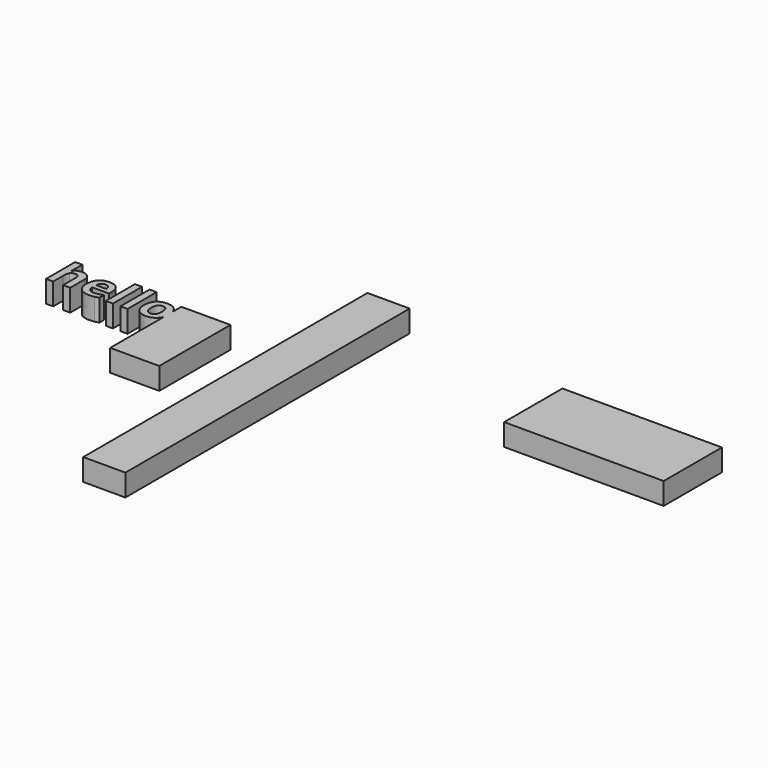
from build123d import *

# Parameters (mm, degrees)
F0_W     = 184.6868768334
F0_H     = 84.2627063394
F0_W_2   = 48.8200113177
F0_H_2   = 411.3924652338
F0_W_3   = 8.2527426776
F0_H_3   = 42.1123689836
F1_DEPTH = 25.4


with BuildPart() as f1:
    # F0 (on Top) → F1 (new body)
    with BuildSketch(Plane.XY):
        with Locations((184.7166828811, 123.0147741735)):
            Rectangle(F0_W, F0_H)
        with Locations((-137.6638747752, -4.5765265822)):
            Rectangle(F0_W_2, F0_H_2)
        with BuildLine():
            Line((-386.5573875373, 41.1865082052), (-378.3046448597, 41.1865082052))
            Line((-378.3046448597, 41.1865082052), (-378.3046448597, 60.9134209226))
            add(Edge.make_bspline(
                [(-381.0627755447, 69.1401843473), (-378.3046448597, 66.2738067751), (-378.3046448597, 60.9134209226)],
                knots=[0, 0, 0, 1, 1, 1], degree=2))
            add(Edge.make_bspline(
                [(-389.1553128293, 72.0065619195), (-383.8209062297, 72.0065619195), (-381.0627755447, 69.1401843473)],
                knots=[0, 0, 0, 1, 1, 1], degree=2))
            add(Edge.make_bspline(
                [(-397.9276405654, 67.5727694211), (-395.1651800049, 72.0065619195), (-389.1553128293, 72.0065619195)],
                knots=[0, 0, 0, 1, 1, 1], degree=2))
            Line((-397.9276405654, 67.5727694211), (-398.3606281141, 67.5727694211))
            Line((-398.3606281141, 67.5727694211), (-398.1701135926, 70.0061594447))
            add(Edge.make_bspline(
                [(-397.9795990712, 74.7170639742), (-397.9795990712, 73.7125328613), (-398.1701135926, 70.0061594447)],
                knots=[0, 0, 0, 1, 1, 1], degree=2))
            Line((-397.9795990712, 74.7170639742), (-397.9795990712, 83.2988771888))
            Line((-397.9795990712, 83.2988771888), (-406.2323417489, 83.2988771888))
            Line((-406.2323417489, 83.2988771888), (-406.2323417489, 41.1865082052))
            Line((-406.2323417489, 41.1865082052), (-397.9795990712, 41.1865082052))
            Line((-397.9795990712, 41.1865082052), (-397.9795990712, 55.4231388055))
            add(Edge.make_bspline(
                [(-396.438163398, 63.052379413), (-397.9795990712, 60.6969271483), (-397.9795990712, 55.4231388055)],
                knots=[0, 0, 0, 1, 1, 1], degree=2))
            add(Edge.make_bspline(
                [(-391.4328273353, 65.4078316778), (-394.8967277247, 65.4078316778), (-396.438163398, 63.052379413)],
                knots=[0, 0, 0, 1, 1, 1], degree=2))
            add(Edge.make_bspline(
                [(-386.5573875373, 58.8610599419), (-386.5573875373, 65.4078316778), (-391.4328273353, 65.4078316778)],
                knots=[0, 0, 0, 1, 1, 1], degree=2))
            Line((-386.5573875373, 58.8610599419), (-386.5573875373, 41.1865082052))
        make_face()
        Polygon((-336.9529306078, 41.1865082052), (-328.8141680467, 41.1865082052), (-328.8141680467, 83.2988771888), (-337.0669107244, 83.2988771888), (-337.0669107244, 41.1865082052), align=None)
        with Locations((-316.0280457345, 62.242692697)):
            Rectangle(F0_W_3, F0_H_3)
        with BuildLine():
            Line((-276.5679955482, 50.2645032945), (-276.5679955482, -28.1147938222))
            Line((-276.5679955482, -28.1147938222), (-219.7534025482, -28.1147938222))
            Line((-219.7534025482, -28.1147938222), (-219.7534025482, 74.9002173543))
            Line((-219.7534025482, 74.9002173543), (-276.5679955482, 74.9002173543))
            Line((-276.5679955482, 74.9002173543), (-276.5679955482, 62.2686307575))
            add(Edge.make_bspline(
                [(-276.5679955482, 62.2686307575), (-275.7472140818, 59.5977436271), (-275.7472140818, 56.3670516616)],
                knots=[0.3216911884, 0.3216911884, 0.3216911884, 1, 1, 1], degree=2))
            add(Edge.make_bspline(
                [(-275.7472140818, 56.3670516616), (-275.7472140818, 52.9769771283), (-276.5679955482, 50.2645032945)],
                knots=[0, 0, 0, 0.4589388385, 0.4589388385, 0.4589388385], degree=2))
        make_face()
        with BuildLine():
            add(Edge.make_bspline(
                [(-356.1183628659, 40.6409438939), (-363.4185329364, 40.6409438939), (-367.5319146488, 44.6763878475)],
                knots=[0, 0, 0, 1, 1, 1], degree=2))
            add(Edge.make_bspline(
                [(-350.1084956903, 41.1691887033), (-352.5678649668, 40.6409438939), (-356.1183628659, 40.6409438939)],
                knots=[0, 0, 0, 1, 1, 1], degree=2))
            add(Edge.make_bspline(
                [(-345.4841886705, 42.7799023843), (-347.6491264139, 41.6974335126), (-350.1084956903, 41.1691887033)],
                knots=[0, 0, 0, 1, 1, 1], degree=2))
            Line((-345.4841886705, 42.7799023843), (-345.4841886705, 49.1707986027))
            add(Edge.make_bspline(
                [(-350.5674624919, 47.3565807737), (-348.1340724684, 47.9237944625), (-345.4841886705, 49.1707986027)],
                knots=[0, 0, 0, 1, 1, 1], degree=2))
            add(Edge.make_bspline(
                [(-355.737333823, 46.789367085), (-353.0008525154, 46.789367085), (-350.5674624919, 47.3565807737)],
                knots=[0, 0, 0, 1, 1, 1], degree=2))
            add(Edge.make_bspline(
                [(-361.2016366872, 48.7637903069), (-359.2531927182, 46.789367085), (-355.737333823, 46.789367085)],
                knots=[0, 0, 0, 1, 1, 1], degree=2))
            add(Edge.make_bspline(
                [(-363.2886366718, 54.2540724241), (-363.1500806562, 50.7382135289), (-361.2016366872, 48.7637903069)],
                knots=[0, 0, 0, 1, 1, 1], degree=2))
            Line((-363.2886366718, 54.2540724241), (-343.7782177288, 54.2540724241))
            Line((-343.7782177288, 54.2540724241), (-343.7782177288, 58.2635371247))
            add(Edge.make_bspline(
                [(-347.3503650053, 68.3564768842), (-343.7782177288, 64.7063918489), (-343.7782177288, 58.2635371247)],
                knots=[0, 0, 0, 1, 1, 1], degree=2))
            add(Edge.make_bspline(
                [(-357.3307280021, 72.0065619195), (-350.9225122818, 72.0065619195), (-347.3503650053, 68.3564768842)],
                knots=[0, 0, 0, 1, 1, 1], degree=2))
            add(Edge.make_bspline(
                [(-367.8436656838, 67.8542113278), (-364.0420350065, 72.0065619195), (-357.3307280021, 72.0065619195)],
                knots=[0, 0, 0, 1, 1, 1], degree=2))
            add(Edge.make_bspline(
                [(-371.6452963611, 56.0985993814), (-371.6452963611, 63.701860736), (-367.8436656838, 67.8542113278)],
                knots=[0, 0, 0, 1, 1, 1], degree=2))
            add(Edge.make_bspline(
                [(-367.5319146488, 44.6763878475), (-371.6452963611, 48.7118318011), (-371.6452963611, 56.0985993814)],
                knots=[0, 0, 0, 1, 1, 1], degree=2))
        make_face()
        with BuildLine():
            add(Edge.make_bspline(
                [(-357.2787694963, 66.1352507595), (-359.9026740412, 66.1352507595), (-361.3921512086, 64.4725785727)],
                knots=[0, 0, 0, 1, 1, 1], degree=2))
            add(Edge.make_bspline(
                [(-353.1134292781, 64.4725785727), (-354.6548649513, 66.1352507595), (-357.2787694963, 66.1352507595)],
                knots=[0, 0, 0, 1, 1, 1], degree=2))
            add(Edge.make_bspline(
                [(-351.511375348, 59.7530142922), (-351.5719936048, 62.8099063858), (-353.1134292781, 64.4725785727)],
                knots=[0, 0, 0, 1, 1, 1], degree=2))
            Line((-351.511375348, 59.7530142922), (-363.0981221504, 59.7530142922))
            add(Edge.make_bspline(
                [(-361.3921512086, 64.4725785727), (-362.8816283761, 62.8099063858), (-363.0981221504, 59.7530142922)],
                knots=[0, 0, 0, 1, 1, 1], degree=2))
        make_face(mode=Mode.SUBTRACT)
        with BuildLine():
            add(Edge.make_bspline(
                [(-276.5679955482, 50.2645032945), (-277.5356473057, 47.0666605317), (-279.6441020198, 44.8106139876)],
                knots=[0.4589388385, 0.4589388385, 0.4589388385, 1, 1, 1], degree=2))
            Line((-276.5679955482, 50.2645032945), (-276.5679955482, 62.2686307575))
            add(Edge.make_bspline(
                [(-277.5311227823, 64.6760827205), (-276.9572550725, 63.5353117149), (-276.5679955482, 62.2686307575)],
                knots=[0, 0, 0, 0.3216911884, 0.3216911884, 0.3216911884], degree=2))
            add(Edge.make_bspline(
                [(-282.6447057321, 70.1144063318), (-279.3150314828, 68.2222507441), (-277.5311227823, 64.6760827205)],
                knots=[0, 0, 0, 1, 1, 1], degree=2))
            add(Edge.make_bspline(
                [(-290.330234721, 72.0065619195), (-285.9743799814, 72.0065619195), (-282.6447057321, 70.1144063318)],
                knots=[0, 0, 0, 1, 1, 1], degree=2))
            add(Edge.make_bspline(
                [(-301.2112118191, 67.8931802071), (-297.3446330094, 72.0065619195), (-290.330234721, 72.0065619195)],
                knots=[0, 0, 0, 1, 1, 1], degree=2))
            add(Edge.make_bspline(
                [(-305.0777906287, 56.3670516616), (-305.0777906287, 63.7797984948), (-301.2112118191, 67.8931802071)],
                knots=[0, 0, 0, 1, 1, 1], degree=2))
            add(Edge.make_bspline(
                [(-303.2938819282, 48.0320413497), (-305.0777906287, 51.6041886262), (-305.0777906287, 56.3670516616)],
                knots=[0, 0, 0, 1, 1, 1], degree=2))
            add(Edge.make_bspline(
                [(-298.1802989784, 42.5504189835), (-301.5099732276, 44.4598940731), (-303.2938819282, 48.0320413497)],
                knots=[0, 0, 0, 1, 1, 1], degree=2))
            add(Edge.make_bspline(
                [(-290.4947699895, 40.6409438939), (-294.8506247291, 40.6409438939), (-298.1802989784, 42.5504189835)],
                knots=[0, 0, 0, 1, 1, 1], degree=2))
            add(Edge.make_bspline(
                [(-279.6441020198, 44.8106139876), (-283.5409899579, 40.6409438939), (-290.4947699895, 40.6409438939)],
                knots=[0, 0, 0, 1, 1, 1], degree=2))
        make_face()
        with BuildLine():
            add(Edge.make_bspline(
                [(-296.6691724335, 56.3670516616), (-296.6691724335, 51.8726409064), (-295.1926848926, 49.5734770229)],
                knots=[0, 0, 0, 1, 1, 1], degree=2))
            add(Edge.make_bspline(
                [(-295.205674519, 63.1216574208), (-296.6691724335, 60.8874416697), (-296.6691724335, 56.3670516616)],
                knots=[0, 0, 0, 1, 1, 1], degree=2))
            add(Edge.make_bspline(
                [(-290.4428114836, 65.3558731719), (-293.7421766045, 65.3558731719), (-295.205674519, 63.1216574208)],
                knots=[0, 0, 0, 1, 1, 1], degree=2))
            add(Edge.make_bspline(
                [(-285.6496393199, 63.1086677943), (-287.1088073589, 65.3558731719), (-290.4428114836, 65.3558731719)],
                knots=[0, 0, 0, 1, 1, 1], degree=2))
            add(Edge.make_bspline(
                [(-284.1904712809, 56.3670516616), (-284.1904712809, 60.8614624167), (-285.6496393199, 63.1086677943)],
                knots=[0, 0, 0, 1, 1, 1], degree=2))
            add(Edge.make_bspline(
                [(-285.6366496934, 49.5604873965), (-284.1904712809, 51.8466616534), (-284.1904712809, 56.3670516616)],
                knots=[0, 0, 0, 1, 1, 1], degree=2))
            add(Edge.make_bspline(
                [(-290.3908529778, 47.2743131395), (-287.082828106, 47.2743131395), (-285.6366496934, 49.5604873965)],
                knots=[0, 0, 0, 1, 1, 1], degree=2))
            add(Edge.make_bspline(
                [(-295.1926848926, 49.5734770229), (-293.7161973516, 47.2743131395), (-290.3908529778, 47.2743131395)],
                knots=[0, 0, 0, 1, 1, 1], degree=2))
        make_face(mode=Mode.SUBTRACT)
        with BuildLine():
            Line((-276.5679955482, 62.2686307575), (-276.5679955482, 50.2645032945))
            add(Edge.make_bspline(
                [(-275.7472140818, 56.3670516616), (-275.7472140818, 52.9769771283), (-276.5679955482, 50.2645032945)],
                knots=[0, 0, 0, 0.4589388385, 0.4589388385, 0.4589388385], degree=2))
            add(Edge.make_bspline(
                [(-276.5679955482, 62.2686307575), (-275.7472140818, 59.5977436271), (-275.7472140818, 56.3670516616)],
                knots=[0.3216911884, 0.3216911884, 0.3216911884, 1, 1, 1], degree=2))
        make_face()
    extrude(amount=F1_DEPTH)


solid = f1.part
